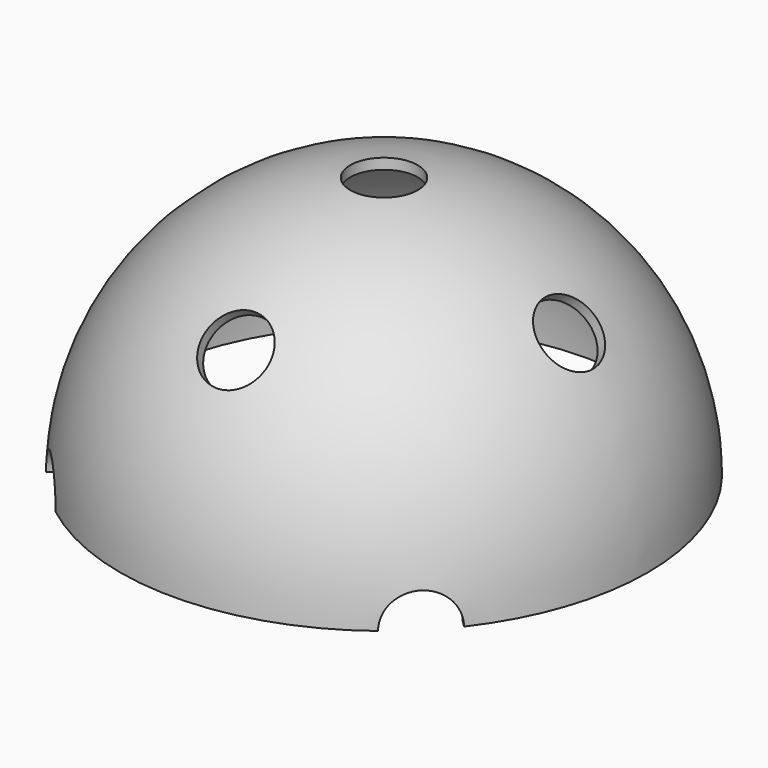
from build123d import *

# Parameters (mm, degrees)
F2_T             = -1
F3_R             = 3.2
F4_DEPTH         = 25.001
F9_R             = 3.2
F10_DEPTH        = 35.3563390593
F10_COPIES_COUNT = 4
F12_R            = 3.2
F13_DEPTH        = 17.6786696004
F15_R            = 3.2
F16_DEPTH        = 17.6786696004
F18_R            = 3.2
F19_DEPTH        = 17.6786696004
F19_DEPTH_BACK   = 25
F19_COPIES_COUNT = 3
F19_COPIES_ANGLE = 180
F21_R            = 3.2
F22_DEPTH        = 17.6786696004
F22_DEPTH_BACK   = 25


# Not quite as in the source:
# - a feature of the source that left no trace in its solid (it failed there, or was rolled back) is left out
# - a pattern or mirror of a feature is missing from the dataset's text; its kind, count and spacing are read off the source's solid


with BuildPart() as f1:
    # F0 (on Front) → F1 (revolve)
    with BuildSketch(Plane.XZ):
        with BuildLine():
            ThreePointArc((25, 0), (17.6776695297, 17.6776695297), (0, 25))
            Line((0, 25), (0, 0))
            Line((0, 0), (25, 0))
        make_face()
    revolve(axis=Axis((0, 0, 12.5), (0, 0, -1)))

    # F2
    f2_openings = [f1.faces().sort_by_distance(p)[0] for p in [
        (0, 0, 0),
    ]]
    offset(amount=F2_T, openings=f2_openings)

    # F3 (on Top) → F4 (cut, through all)
    with BuildSketch(Plane.XY):
        Circle(F3_R)
    extrude(amount=F4_DEPTH, mode=Mode.SUBTRACT)

    # F9 (on face) → F10 (cut, through all)
    with BuildSketch(Plane(origin=(0, 0, 0), x_dir=(0.7071067812, -0.7071067812, 0), z_dir=(-0.7071067812, -0.7071067812, 0))):
        Circle(F9_R)
    f10 = extrude(amount=-F10_DEPTH, mode=Mode.SUBTRACT)

    # F10_copies: F10 ×4 about axis
    f10_copies_axis = Axis((0, 0, 0), (0, 0, 1))
    for i in range(1, F10_COPIES_COUNT):
        add(f10.rotate(f10_copies_axis, i * 360 / F10_COPIES_COUNT), mode=Mode.SUBTRACT)

    # F12 (on face) → F13 (cut, through all)
    with BuildSketch(Plane(origin=(0, 0, 0), x_dir=(0, 1, 0), z_dir=(0.7071067812, 0, -0.7071067812))):
        Circle(F12_R)
    extrude(amount=F13_DEPTH, mode=Mode.SUBTRACT)

    # F15 (on face) → F16 (cut, through all)
    with BuildSketch(Plane(origin=(0, 0, 0), x_dir=(1, 0, 0), z_dir=(0, -0.7071067812, -0.7071067812))):
        Circle(F15_R)
    extrude(amount=F16_DEPTH, mode=Mode.SUBTRACT)

    # F18 (on face) → F19 (cut, two sides)
    with BuildSketch(Plane(origin=(0, 0, 0), x_dir=(0, 1, 0), z_dir=(0.7071067812, 0, 0.7071067812))) as f19_sk:
        Circle(F18_R)
    f19 = extrude(amount=-F19_DEPTH, mode=Mode.SUBTRACT) + extrude(f19_sk.sketch, amount=F19_DEPTH_BACK, mode=Mode.SUBTRACT)

    # F19_copies: F19 ×3 about axis
    f19_copies_axis = Axis((0, 0, 0), (0, 0, 1))
    for i in range(1, F19_COPIES_COUNT):
        add(f19.rotate(f19_copies_axis, i * F19_COPIES_ANGLE / (F19_COPIES_COUNT - 1)), mode=Mode.SUBTRACT)

    # F21 (on face) → F22 (cut, two sides)
    with BuildSketch(Plane(origin=(0, 0, 0), x_dir=(1, 0, 0), z_dir=(0, -0.7071067812, 0.7071067812))) as f22_sk:
        Circle(F21_R)
    extrude(amount=-F22_DEPTH, mode=Mode.SUBTRACT)
    extrude(f22_sk.sketch, amount=F22_DEPTH_BACK, mode=Mode.SUBTRACT)


solid = f1.part
